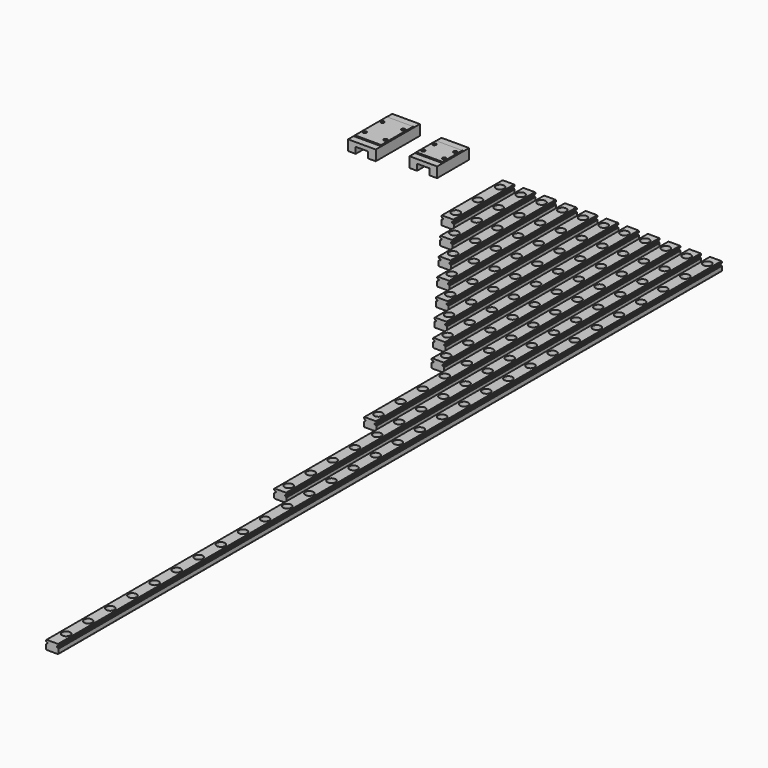
from build123d import *

# Parameters (mm, degrees)
F1_DEPTH           = 55
F2_DEPTH           = 75
F3_DEPTH           = 95
F4_DEPTH           = 115
F5_DEPTH           = 135
F6_DEPTH           = 155
F7_DEPTH           = 175
F8_DEPTH           = 195
F9_DEPTH           = 275
F10_DEPTH          = 375
F11_DEPTH          = 600
F13_D              = 3.5
F13_CBORE_D        = 6
F13_CBORE_DEPTH    = 3.5
F13_2_D            = 3.5
F13_2_CBORE_D      = 6
F13_2_CBORE_DEPTH  = 3.5
F13_3_D            = 3.5
F13_3_CBORE_D      = 6
F13_3_CBORE_DEPTH  = 3.5
F13_4_D            = 3.5
F13_4_CBORE_D      = 6
F13_4_CBORE_DEPTH  = 3.5
F13_5_D            = 3.5
F13_5_CBORE_D      = 6
F13_5_CBORE_DEPTH  = 3.5
F13_6_D            = 3.5
F13_6_CBORE_D      = 6
F13_6_CBORE_DEPTH  = 3.5
F13_7_D            = 3.5
F13_7_CBORE_D      = 6
F13_7_CBORE_DEPTH  = 3.5
F13_8_D            = 3.5
F13_8_CBORE_D      = 6
F13_8_CBORE_DEPTH  = 3.5
F13_9_D            = 3.5
F13_9_CBORE_D      = 6
F13_9_CBORE_DEPTH  = 3.5
F13_10_D           = 3.5
F13_10_CBORE_D     = 6
F13_10_CBORE_DEPTH = 3.5
F14_D              = 3.5
F14_CBORE_D        = 6
F14_CBORE_DEPTH    = 3.5
F16_DEPTH          = 9.45
F18_DEPTH          = 5
F19_DEPTH          = 14.95
F21_DEPTH          = 5
F23_D              = 2.5
F23_DEPTH          = 4.1
F23_TIP            = 0.7510757738
F23_2_D            = 2.5
F23_2_DEPTH        = 4.1
F23_2_TIP          = 0.7510757738
F25_SIZE           = 0.49999


# Not quite as in the source:
# - a fillet or chamfer is up to 0.001 mm smaller than in the source, because OpenCascade refuses the exact size


with BuildPart() as f1:
    # F0 (on Front) → F1 (new body)
    with BuildSketch(Plane.XZ):
        with BuildLine():
            Line((-4.1464466094, -3.25), (4.1464466094, -3.25))
            Line((4.1464466094, -3.25), (4.5, -2.8964466094))
            Line((4.5, -2.8964466094), (4.5, 0.2817541634))
            ThreePointArc((4.5, 0.2817541634), (4.1012202029, 0.4890238013), (3.833484861, 0.85))
            Line((3.833484861, 0.85), (3.3, 0.85))
            Line((3.3, 0.85), (3.3, 1.65))
            Line((3.3, 1.65), (3.833484861, 1.65))
            ThreePointArc((3.833484861, 1.65), (4.1012202029, 2.0109761987), (4.5, 2.2182458366))
            Line((4.5, 2.2182458366), (4.5, 2.8964466094))
            Line((4.5, 2.8964466094), (4.1464466094, 3.25))
            Line((4.1464466094, 3.25), (-4.1464466094, 3.25))
            Line((-4.1464466094, 3.25), (-4.5, 2.8964466094))
            Line((-4.5, 2.8964466094), (-4.5, 2.2182458366))
            ThreePointArc((-4.5, 2.2182458366), (-4.1012202029, 2.0109761987), (-3.833484861, 1.65))
            Line((-3.833484861, 1.65), (-3.3, 1.65))
            Line((-3.3, 1.65), (-3.3, 0.85))
            Line((-3.3, 0.85), (-3.833484861, 0.85))
            ThreePointArc((-3.833484861, 0.85), (-4.1012202029, 0.4890238013), (-4.5, 0.2817541634))
            Line((-4.5, 0.2817541634), (-4.5, -2.8964466094))
            Line((-4.5, -2.8964466094), (-4.1464466094, -3.25))
        make_face()
    extrude(amount=F1_DEPTH)

    # F13 (through all)
    with Locations(Plane.XY.offset(3.25)):
        with Locations((75, -7.5), (135, -47.5), (15, -47.5), (60, -7.5), (90, -27.5), (90, -47.5), (120, -27.5), (30, -7.5), (105, -7.5), (30, -47.5), (0, -47.5), (75, -47.5), (45, -7.5), (90, -7.5), (120, -47.5), (105, -27.5), (15, -7.5), (105, -47.5), (75, -27.5), (135, -27.5), (45, -47.5), (0, -7.5), (60, -47.5), (30, -27.5), (120, -7.5), (45, -27.5), (135, -7.5), (60, -27.5), (0, -27.5), (15, -27.5), (135, -67.5), (30, -67.5), (120, -67.5), (45, -67.5), (15, -67.5), (105, -67.5), (60, -67.5), (75, -67.5), (90, -67.5), (30, -87.5), (45, -87.5), (75, -87.5), (60, -87.5), (105, -87.5), (90, -87.5), (135, -87.5), (120, -87.5), (75, -107.5), (45, -107.5), (60, -107.5), (135, -107.5), (105, -107.5), (120, -107.5), (90, -107.5), (135, -127.5), (105, -127.5), (120, -127.5), (60, -127.5), (75, -127.5), (90, -127.5), (75, -147.5), (90, -147.5), (120, -147.5), (105, -147.5), (135, -147.5), (90, -167.5), (105, -167.5), (135, -167.5), (120, -167.5), (135, -187.5), (105, -187.5), (120, -187.5), (120, -227.5), (135, -267.5), (135, -227.5), (120, -267.5), (120, -207.5), (135, -207.5), (135, -247.5), (120, -247.5), (135, -307.5), (135, -347.5), (135, -367.5), (135, -327.5), (135, -287.5)):
            CounterBoreHole(F13_D / 2, F13_CBORE_D / 2, F13_CBORE_DEPTH)


with BuildPart() as f2:
    # F0 (on Front) → F2 (new body)
    with BuildSketch(Plane.XZ):
        with BuildLine():
            Line((10.5, 0.2817541634), (10.5, -2.8964466094))
            Line((10.5, -2.8964466094), (10.8535533906, -3.25))
            Line((10.8535533906, -3.25), (19.1464466094, -3.25))
            Line((19.1464466094, -3.25), (19.5, -2.8964466094))
            Line((19.5, -2.8964466094), (19.5, 0.2817541634))
            ThreePointArc((19.5, 0.2817541634), (19.1012202029, 0.4890238013), (18.833484861, 0.85))
            Line((18.833484861, 0.85), (18.3, 0.85))
            Line((18.3, 0.85), (18.3, 1.65))
            Line((18.3, 1.65), (18.833484861, 1.65))
            ThreePointArc((18.833484861, 1.65), (19.1012202029, 2.0109761987), (19.5, 2.2182458366))
            Line((19.5, 2.2182458366), (19.5, 2.8964466094))
            Line((19.5, 2.8964466094), (19.1464466094, 3.25))
            Line((19.1464466094, 3.25), (10.8535533906, 3.25))
            Line((10.8535533906, 3.25), (10.5, 2.8964466094))
            Line((10.5, 2.8964466094), (10.5, 2.2182458366))
            ThreePointArc((10.5, 2.2182458366), (10.8987797971, 2.0109761987), (11.166515139, 1.65))
            Line((11.166515139, 1.65), (11.7, 1.65))
            Line((11.7, 1.65), (11.7, 0.85))
            Line((11.7, 0.85), (11.166515139, 0.85))
            ThreePointArc((11.166515139, 0.85), (10.8987797971, 0.4890238013), (10.5, 0.2817541634))
        make_face()
    extrude(amount=F2_DEPTH)

    # F13#2 (through all)
    with Locations(Plane.XY.offset(3.25)):
        with Locations((75, -7.5), (135, -47.5), (15, -47.5), (60, -7.5), (90, -27.5), (90, -47.5), (120, -27.5), (30, -7.5), (105, -7.5), (30, -47.5), (0, -47.5), (75, -47.5), (45, -7.5), (90, -7.5), (120, -47.5), (105, -27.5), (15, -7.5), (105, -47.5), (75, -27.5), (135, -27.5), (45, -47.5), (0, -7.5), (60, -47.5), (30, -27.5), (120, -7.5), (45, -27.5), (135, -7.5), (60, -27.5), (0, -27.5), (15, -27.5), (135, -67.5), (30, -67.5), (120, -67.5), (45, -67.5), (15, -67.5), (105, -67.5), (60, -67.5), (75, -67.5), (90, -67.5), (30, -87.5), (45, -87.5), (75, -87.5), (60, -87.5), (105, -87.5), (90, -87.5), (135, -87.5), (120, -87.5), (75, -107.5), (45, -107.5), (60, -107.5), (135, -107.5), (105, -107.5), (120, -107.5), (90, -107.5), (135, -127.5), (105, -127.5), (120, -127.5), (60, -127.5), (75, -127.5), (90, -127.5), (75, -147.5), (90, -147.5), (120, -147.5), (105, -147.5), (135, -147.5), (90, -167.5), (105, -167.5), (135, -167.5), (120, -167.5), (135, -187.5), (105, -187.5), (120, -187.5), (120, -227.5), (135, -267.5), (135, -227.5), (120, -267.5), (120, -207.5), (135, -207.5), (135, -247.5), (120, -247.5), (135, -307.5), (135, -347.5), (135, -367.5), (135, -327.5), (135, -287.5)):
            CounterBoreHole(F13_2_D / 2, F13_2_CBORE_D / 2, F13_2_CBORE_DEPTH)


with BuildPart() as f3:
    # F0 (on Front) → F3 (new body)
    with BuildSketch(Plane.XZ):
        with BuildLine():
            Line((25.5, 0.2817541634), (25.5, -2.8964466094))
            Line((25.5, -2.8964466094), (25.8535533906, -3.25))
            Line((25.8535533906, -3.25), (34.1464466094, -3.25))
            Line((34.1464466094, -3.25), (34.5, -2.8964466094))
            Line((34.5, -2.8964466094), (34.5, 0.2817541634))
            ThreePointArc((34.5, 0.2817541634), (34.1012202029, 0.4890238013), (33.833484861, 0.85))
            Line((33.833484861, 0.85), (33.3, 0.85))
            Line((33.3, 0.85), (33.3, 1.65))
            Line((33.3, 1.65), (33.833484861, 1.65))
            ThreePointArc((33.833484861, 1.65), (34.1012202029, 2.0109761987), (34.5, 2.2182458366))
            Line((34.5, 2.2182458366), (34.5, 2.8964466094))
            Line((34.5, 2.8964466094), (34.1464466094, 3.25))
            Line((34.1464466094, 3.25), (25.8535533906, 3.25))
            Line((25.8535533906, 3.25), (25.5, 2.8964466094))
            Line((25.5, 2.8964466094), (25.5, 2.2182458366))
            ThreePointArc((25.5, 2.2182458366), (25.8987797971, 2.0109761987), (26.166515139, 1.65))
            Line((26.166515139, 1.65), (26.7, 1.65))
            Line((26.7, 1.65), (26.7, 0.85))
            Line((26.7, 0.85), (26.166515139, 0.85))
            ThreePointArc((26.166515139, 0.85), (25.8987797971, 0.4890238013), (25.5, 0.2817541634))
        make_face()
    extrude(amount=F3_DEPTH)

    # F13#3 (through all)
    with Locations(Plane.XY.offset(3.25)):
        with Locations((75, -7.5), (135, -47.5), (15, -47.5), (60, -7.5), (90, -27.5), (90, -47.5), (120, -27.5), (30, -7.5), (105, -7.5), (30, -47.5), (0, -47.5), (75, -47.5), (45, -7.5), (90, -7.5), (120, -47.5), (105, -27.5), (15, -7.5), (105, -47.5), (75, -27.5), (135, -27.5), (45, -47.5), (0, -7.5), (60, -47.5), (30, -27.5), (120, -7.5), (45, -27.5), (135, -7.5), (60, -27.5), (0, -27.5), (15, -27.5), (135, -67.5), (30, -67.5), (120, -67.5), (45, -67.5), (15, -67.5), (105, -67.5), (60, -67.5), (75, -67.5), (90, -67.5), (30, -87.5), (45, -87.5), (75, -87.5), (60, -87.5), (105, -87.5), (90, -87.5), (135, -87.5), (120, -87.5), (75, -107.5), (45, -107.5), (60, -107.5), (135, -107.5), (105, -107.5), (120, -107.5), (90, -107.5), (135, -127.5), (105, -127.5), (120, -127.5), (60, -127.5), (75, -127.5), (90, -127.5), (75, -147.5), (90, -147.5), (120, -147.5), (105, -147.5), (135, -147.5), (90, -167.5), (105, -167.5), (135, -167.5), (120, -167.5), (135, -187.5), (105, -187.5), (120, -187.5), (120, -227.5), (135, -267.5), (135, -227.5), (120, -267.5), (120, -207.5), (135, -207.5), (135, -247.5), (120, -247.5), (135, -307.5), (135, -347.5), (135, -367.5), (135, -327.5), (135, -287.5)):
            CounterBoreHole(F13_3_D / 2, F13_3_CBORE_D / 2, F13_3_CBORE_DEPTH)


with BuildPart() as f4:
    # F0 (on Front) → F4 (new body)
    with BuildSketch(Plane.XZ):
        with BuildLine():
            Line((40.5, 0.2817541634), (40.5, -2.8964466094))
            Line((40.5, -2.8964466094), (40.8535533906, -3.25))
            Line((40.8535533906, -3.25), (49.1464466094, -3.25))
            Line((49.1464466094, -3.25), (49.5, -2.8964466094))
            Line((49.5, -2.8964466094), (49.5, 0.2817541634))
            ThreePointArc((49.5, 0.2817541634), (49.1012202029, 0.4890238013), (48.833484861, 0.85))
            Line((48.833484861, 0.85), (48.3, 0.85))
            Line((48.3, 0.85), (48.3, 1.65))
            Line((48.3, 1.65), (48.833484861, 1.65))
            ThreePointArc((48.833484861, 1.65), (49.1012202029, 2.0109761987), (49.5, 2.2182458366))
            Line((49.5, 2.2182458366), (49.5, 2.8964466094))
            Line((49.5, 2.8964466094), (49.1464466094, 3.25))
            Line((49.1464466094, 3.25), (40.8535533906, 3.25))
            Line((40.8535533906, 3.25), (40.5, 2.8964466094))
            Line((40.5, 2.8964466094), (40.5, 2.2182458366))
            ThreePointArc((40.5, 2.2182458366), (40.8987797971, 2.0109761987), (41.166515139, 1.65))
            Line((41.166515139, 1.65), (41.7, 1.65))
            Line((41.7, 1.65), (41.7, 0.85))
            Line((41.7, 0.85), (41.166515139, 0.85))
            ThreePointArc((41.166515139, 0.85), (40.8987797971, 0.4890238013), (40.5, 0.2817541634))
        make_face()
    extrude(amount=F4_DEPTH)

    # F13#4 (through all)
    with Locations(Plane.XY.offset(3.25)):
        with Locations((75, -7.5), (135, -47.5), (15, -47.5), (60, -7.5), (90, -27.5), (90, -47.5), (120, -27.5), (30, -7.5), (105, -7.5), (30, -47.5), (0, -47.5), (75, -47.5), (45, -7.5), (90, -7.5), (120, -47.5), (105, -27.5), (15, -7.5), (105, -47.5), (75, -27.5), (135, -27.5), (45, -47.5), (0, -7.5), (60, -47.5), (30, -27.5), (120, -7.5), (45, -27.5), (135, -7.5), (60, -27.5), (0, -27.5), (15, -27.5), (135, -67.5), (30, -67.5), (120, -67.5), (45, -67.5), (15, -67.5), (105, -67.5), (60, -67.5), (75, -67.5), (90, -67.5), (30, -87.5), (45, -87.5), (75, -87.5), (60, -87.5), (105, -87.5), (90, -87.5), (135, -87.5), (120, -87.5), (75, -107.5), (45, -107.5), (60, -107.5), (135, -107.5), (105, -107.5), (120, -107.5), (90, -107.5), (135, -127.5), (105, -127.5), (120, -127.5), (60, -127.5), (75, -127.5), (90, -127.5), (75, -147.5), (90, -147.5), (120, -147.5), (105, -147.5), (135, -147.5), (90, -167.5), (105, -167.5), (135, -167.5), (120, -167.5), (135, -187.5), (105, -187.5), (120, -187.5), (120, -227.5), (135, -267.5), (135, -227.5), (120, -267.5), (120, -207.5), (135, -207.5), (135, -247.5), (120, -247.5), (135, -307.5), (135, -347.5), (135, -367.5), (135, -327.5), (135, -287.5)):
            CounterBoreHole(F13_4_D / 2, F13_4_CBORE_D / 2, F13_4_CBORE_DEPTH)


with BuildPart() as f5:
    # F0 (on Front) → F5 (new body)
    with BuildSketch(Plane.XZ):
        with BuildLine():
            Line((55.5, 0.2817541634), (55.5, -2.8964466094))
            Line((55.5, -2.8964466094), (55.8535533906, -3.25))
            Line((55.8535533906, -3.25), (64.1464466094, -3.25))
            Line((64.1464466094, -3.25), (64.5, -2.8964466094))
            Line((64.5, -2.8964466094), (64.5, 0.2817541634))
            ThreePointArc((64.5, 0.2817541634), (64.1012202029, 0.4890238013), (63.833484861, 0.85))
            Line((63.833484861, 0.85), (63.3, 0.85))
            Line((63.3, 0.85), (63.3, 1.65))
            Line((63.3, 1.65), (63.833484861, 1.65))
            ThreePointArc((63.833484861, 1.65), (64.1012202029, 2.0109761987), (64.5, 2.2182458366))
            Line((64.5, 2.2182458366), (64.5, 2.8964466094))
            Line((64.5, 2.8964466094), (64.1464466094, 3.25))
            Line((64.1464466094, 3.25), (55.8535533906, 3.25))
            Line((55.8535533906, 3.25), (55.5, 2.8964466094))
            Line((55.5, 2.8964466094), (55.5, 2.2182458366))
            ThreePointArc((55.5, 2.2182458366), (55.8987797971, 2.0109761987), (56.166515139, 1.65))
            Line((56.166515139, 1.65), (56.7, 1.65))
            Line((56.7, 1.65), (56.7, 0.85))
            Line((56.7, 0.85), (56.166515139, 0.85))
            ThreePointArc((56.166515139, 0.85), (55.8987797971, 0.4890238013), (55.5, 0.2817541634))
        make_face()
    extrude(amount=F5_DEPTH)

    # F13#5 (through all)
    with Locations(Plane.XY.offset(3.25)):
        with Locations((75, -7.5), (135, -47.5), (15, -47.5), (60, -7.5), (90, -27.5), (90, -47.5), (120, -27.5), (30, -7.5), (105, -7.5), (30, -47.5), (0, -47.5), (75, -47.5), (45, -7.5), (90, -7.5), (120, -47.5), (105, -27.5), (15, -7.5), (105, -47.5), (75, -27.5), (135, -27.5), (45, -47.5), (0, -7.5), (60, -47.5), (30, -27.5), (120, -7.5), (45, -27.5), (135, -7.5), (60, -27.5), (0, -27.5), (15, -27.5), (135, -67.5), (30, -67.5), (120, -67.5), (45, -67.5), (15, -67.5), (105, -67.5), (60, -67.5), (75, -67.5), (90, -67.5), (30, -87.5), (45, -87.5), (75, -87.5), (60, -87.5), (105, -87.5), (90, -87.5), (135, -87.5), (120, -87.5), (75, -107.5), (45, -107.5), (60, -107.5), (135, -107.5), (105, -107.5), (120, -107.5), (90, -107.5), (135, -127.5), (105, -127.5), (120, -127.5), (60, -127.5), (75, -127.5), (90, -127.5), (75, -147.5), (90, -147.5), (120, -147.5), (105, -147.5), (135, -147.5), (90, -167.5), (105, -167.5), (135, -167.5), (120, -167.5), (135, -187.5), (105, -187.5), (120, -187.5), (120, -227.5), (135, -267.5), (135, -227.5), (120, -267.5), (120, -207.5), (135, -207.5), (135, -247.5), (120, -247.5), (135, -307.5), (135, -347.5), (135, -367.5), (135, -327.5), (135, -287.5)):
            CounterBoreHole(F13_5_D / 2, F13_5_CBORE_D / 2, F13_5_CBORE_DEPTH)


with BuildPart() as f6:
    # F0 (on Front) → F6 (new body)
    with BuildSketch(Plane.XZ):
        with BuildLine():
            Line((70.5, 0.2817541634), (70.5, -2.8964466094))
            Line((70.5, -2.8964466094), (70.8535533906, -3.25))
            Line((70.8535533906, -3.25), (79.1464466094, -3.25))
            Line((79.1464466094, -3.25), (79.5, -2.8964466094))
            Line((79.5, -2.8964466094), (79.5, 0.2817541634))
            ThreePointArc((79.5, 0.2817541634), (79.1012202029, 0.4890238013), (78.833484861, 0.85))
            Line((78.833484861, 0.85), (78.3, 0.85))
            Line((78.3, 0.85), (78.3, 1.65))
            Line((78.3, 1.65), (78.833484861, 1.65))
            ThreePointArc((78.833484861, 1.65), (79.1012202029, 2.0109761987), (79.5, 2.2182458366))
            Line((79.5, 2.2182458366), (79.5, 2.8964466094))
            Line((79.5, 2.8964466094), (79.1464466094, 3.25))
            Line((79.1464466094, 3.25), (70.8535533906, 3.25))
            Line((70.8535533906, 3.25), (70.5, 2.8964466094))
            Line((70.5, 2.8964466094), (70.5, 2.2182458366))
            ThreePointArc((70.5, 2.2182458366), (70.8987797971, 2.0109761987), (71.166515139, 1.65))
            Line((71.166515139, 1.65), (71.7, 1.65))
            Line((71.7, 1.65), (71.7, 0.85))
            Line((71.7, 0.85), (71.166515139, 0.85))
            ThreePointArc((71.166515139, 0.85), (70.8987797971, 0.4890238013), (70.5, 0.2817541634))
        make_face()
    extrude(amount=F6_DEPTH)

    # F13#6 (through all)
    with Locations(Plane.XY.offset(3.25)):
        with Locations((75, -7.5), (135, -47.5), (15, -47.5), (60, -7.5), (90, -27.5), (90, -47.5), (120, -27.5), (30, -7.5), (105, -7.5), (30, -47.5), (0, -47.5), (75, -47.5), (45, -7.5), (90, -7.5), (120, -47.5), (105, -27.5), (15, -7.5), (105, -47.5), (75, -27.5), (135, -27.5), (45, -47.5), (0, -7.5), (60, -47.5), (30, -27.5), (120, -7.5), (45, -27.5), (135, -7.5), (60, -27.5), (0, -27.5), (15, -27.5), (135, -67.5), (30, -67.5), (120, -67.5), (45, -67.5), (15, -67.5), (105, -67.5), (60, -67.5), (75, -67.5), (90, -67.5), (30, -87.5), (45, -87.5), (75, -87.5), (60, -87.5), (105, -87.5), (90, -87.5), (135, -87.5), (120, -87.5), (75, -107.5), (45, -107.5), (60, -107.5), (135, -107.5), (105, -107.5), (120, -107.5), (90, -107.5), (135, -127.5), (105, -127.5), (120, -127.5), (60, -127.5), (75, -127.5), (90, -127.5), (75, -147.5), (90, -147.5), (120, -147.5), (105, -147.5), (135, -147.5), (90, -167.5), (105, -167.5), (135, -167.5), (120, -167.5), (135, -187.5), (105, -187.5), (120, -187.5), (120, -227.5), (135, -267.5), (135, -227.5), (120, -267.5), (120, -207.5), (135, -207.5), (135, -247.5), (120, -247.5), (135, -307.5), (135, -347.5), (135, -367.5), (135, -327.5), (135, -287.5)):
            CounterBoreHole(F13_6_D / 2, F13_6_CBORE_D / 2, F13_6_CBORE_DEPTH)


with BuildPart() as f7:
    # F0 (on Front) → F7 (new body)
    with BuildSketch(Plane.XZ):
        with BuildLine():
            Line((85.5, 0.2817541634), (85.5, -2.8964466094))
            Line((85.5, -2.8964466094), (85.8535533906, -3.25))
            Line((85.8535533906, -3.25), (94.1464466094, -3.25))
            Line((94.1464466094, -3.25), (94.5, -2.8964466094))
            Line((94.5, -2.8964466094), (94.5, 0.2817541634))
            ThreePointArc((94.5, 0.2817541634), (94.1012202029, 0.4890238013), (93.833484861, 0.85))
            Line((93.833484861, 0.85), (93.3, 0.85))
            Line((93.3, 0.85), (93.3, 1.65))
            Line((93.3, 1.65), (93.833484861, 1.65))
            ThreePointArc((93.833484861, 1.65), (94.1012202029, 2.0109761987), (94.5, 2.2182458366))
            Line((94.5, 2.2182458366), (94.5, 2.8964466094))
            Line((94.5, 2.8964466094), (94.1464466094, 3.25))
            Line((94.1464466094, 3.25), (85.8535533906, 3.25))
            Line((85.8535533906, 3.25), (85.5, 2.8964466094))
            Line((85.5, 2.8964466094), (85.5, 2.2182458366))
            ThreePointArc((85.5, 2.2182458366), (85.8987797971, 2.0109761987), (86.166515139, 1.65))
            Line((86.166515139, 1.65), (86.7, 1.65))
            Line((86.7, 1.65), (86.7, 0.85))
            Line((86.7, 0.85), (86.166515139, 0.85))
            ThreePointArc((86.166515139, 0.85), (85.8987797971, 0.4890238013), (85.5, 0.2817541634))
        make_face()
    extrude(amount=F7_DEPTH)

    # F13#7 (through all)
    with Locations(Plane.XY.offset(3.25)):
        with Locations((75, -7.5), (135, -47.5), (15, -47.5), (60, -7.5), (90, -27.5), (90, -47.5), (120, -27.5), (30, -7.5), (105, -7.5), (30, -47.5), (0, -47.5), (75, -47.5), (45, -7.5), (90, -7.5), (120, -47.5), (105, -27.5), (15, -7.5), (105, -47.5), (75, -27.5), (135, -27.5), (45, -47.5), (0, -7.5), (60, -47.5), (30, -27.5), (120, -7.5), (45, -27.5), (135, -7.5), (60, -27.5), (0, -27.5), (15, -27.5), (135, -67.5), (30, -67.5), (120, -67.5), (45, -67.5), (15, -67.5), (105, -67.5), (60, -67.5), (75, -67.5), (90, -67.5), (30, -87.5), (45, -87.5), (75, -87.5), (60, -87.5), (105, -87.5), (90, -87.5), (135, -87.5), (120, -87.5), (75, -107.5), (45, -107.5), (60, -107.5), (135, -107.5), (105, -107.5), (120, -107.5), (90, -107.5), (135, -127.5), (105, -127.5), (120, -127.5), (60, -127.5), (75, -127.5), (90, -127.5), (75, -147.5), (90, -147.5), (120, -147.5), (105, -147.5), (135, -147.5), (90, -167.5), (105, -167.5), (135, -167.5), (120, -167.5), (135, -187.5), (105, -187.5), (120, -187.5), (120, -227.5), (135, -267.5), (135, -227.5), (120, -267.5), (120, -207.5), (135, -207.5), (135, -247.5), (120, -247.5), (135, -307.5), (135, -347.5), (135, -367.5), (135, -327.5), (135, -287.5)):
            CounterBoreHole(F13_7_D / 2, F13_7_CBORE_D / 2, F13_7_CBORE_DEPTH)


with BuildPart() as f8:
    # F0 (on Front) → F8 (new body)
    with BuildSketch(Plane.XZ):
        with BuildLine():
            Line((100.5, 0.2817541634), (100.5, -2.8964466094))
            Line((100.5, -2.8964466094), (100.8535533906, -3.25))
            Line((100.8535533906, -3.25), (109.1464466094, -3.25))
            Line((109.1464466094, -3.25), (109.5, -2.8964466094))
            Line((109.5, -2.8964466094), (109.5, 0.2817541634))
            ThreePointArc((109.5, 0.2817541634), (109.1012202029, 0.4890238013), (108.833484861, 0.85))
            Line((108.833484861, 0.85), (108.3, 0.85))
            Line((108.3, 0.85), (108.3, 1.65))
            Line((108.3, 1.65), (108.833484861, 1.65))
            ThreePointArc((108.833484861, 1.65), (109.1012202029, 2.0109761987), (109.5, 2.2182458366))
            Line((109.5, 2.2182458366), (109.5, 2.8964466094))
            Line((109.5, 2.8964466094), (109.1464466094, 3.25))
            Line((109.1464466094, 3.25), (100.8535533906, 3.25))
            Line((100.8535533906, 3.25), (100.5, 2.8964466094))
            Line((100.5, 2.8964466094), (100.5, 2.2182458366))
            ThreePointArc((100.5, 2.2182458366), (100.8987797971, 2.0109761987), (101.166515139, 1.65))
            Line((101.166515139, 1.65), (101.7, 1.65))
            Line((101.7, 1.65), (101.7, 0.85))
            Line((101.7, 0.85), (101.166515139, 0.85))
            ThreePointArc((101.166515139, 0.85), (100.8987797971, 0.4890238013), (100.5, 0.2817541634))
        make_face()
    extrude(amount=F8_DEPTH)

    # F13#8 (through all)
    with Locations(Plane.XY.offset(3.25)):
        with Locations((75, -7.5), (135, -47.5), (15, -47.5), (60, -7.5), (90, -27.5), (90, -47.5), (120, -27.5), (30, -7.5), (105, -7.5), (30, -47.5), (0, -47.5), (75, -47.5), (45, -7.5), (90, -7.5), (120, -47.5), (105, -27.5), (15, -7.5), (105, -47.5), (75, -27.5), (135, -27.5), (45, -47.5), (0, -7.5), (60, -47.5), (30, -27.5), (120, -7.5), (45, -27.5), (135, -7.5), (60, -27.5), (0, -27.5), (15, -27.5), (135, -67.5), (30, -67.5), (120, -67.5), (45, -67.5), (15, -67.5), (105, -67.5), (60, -67.5), (75, -67.5), (90, -67.5), (30, -87.5), (45, -87.5), (75, -87.5), (60, -87.5), (105, -87.5), (90, -87.5), (135, -87.5), (120, -87.5), (75, -107.5), (45, -107.5), (60, -107.5), (135, -107.5), (105, -107.5), (120, -107.5), (90, -107.5), (135, -127.5), (105, -127.5), (120, -127.5), (60, -127.5), (75, -127.5), (90, -127.5), (75, -147.5), (90, -147.5), (120, -147.5), (105, -147.5), (135, -147.5), (90, -167.5), (105, -167.5), (135, -167.5), (120, -167.5), (135, -187.5), (105, -187.5), (120, -187.5), (120, -227.5), (135, -267.5), (135, -227.5), (120, -267.5), (120, -207.5), (135, -207.5), (135, -247.5), (120, -247.5), (135, -307.5), (135, -347.5), (135, -367.5), (135, -327.5), (135, -287.5)):
            CounterBoreHole(F13_8_D / 2, F13_8_CBORE_D / 2, F13_8_CBORE_DEPTH)


with BuildPart() as f9:
    # F0 (on Front) → F9 (new body)
    with BuildSketch(Plane.XZ):
        with BuildLine():
            Line((115.5, 0.2817541634), (115.5, -2.8964466094))
            Line((115.5, -2.8964466094), (115.8535533906, -3.25))
            Line((115.8535533906, -3.25), (124.1464466094, -3.25))
            Line((124.1464466094, -3.25), (124.5, -2.8964466094))
            Line((124.5, -2.8964466094), (124.5, 0.2817541634))
            ThreePointArc((124.5, 0.2817541634), (124.1012202029, 0.4890238013), (123.833484861, 0.85))
            Line((123.833484861, 0.85), (123.3, 0.85))
            Line((123.3, 0.85), (123.3, 1.65))
            Line((123.3, 1.65), (123.833484861, 1.65))
            ThreePointArc((123.833484861, 1.65), (124.1012202029, 2.0109761987), (124.5, 2.2182458366))
            Line((124.5, 2.2182458366), (124.5, 2.8964466094))
            Line((124.5, 2.8964466094), (124.1464466094, 3.25))
            Line((124.1464466094, 3.25), (115.8535533906, 3.25))
            Line((115.8535533906, 3.25), (115.5, 2.8964466094))
            Line((115.5, 2.8964466094), (115.5, 2.2182458366))
            ThreePointArc((115.5, 2.2182458366), (115.8987797971, 2.0109761987), (116.166515139, 1.65))
            Line((116.166515139, 1.65), (116.7, 1.65))
            Line((116.7, 1.65), (116.7, 0.85))
            Line((116.7, 0.85), (116.166515139, 0.85))
            ThreePointArc((116.166515139, 0.85), (115.8987797971, 0.4890238013), (115.5, 0.2817541634))
        make_face()
    extrude(amount=F9_DEPTH)

    # F13#9 (through all)
    with Locations(Plane.XY.offset(3.25)):
        with Locations((75, -7.5), (135, -47.5), (15, -47.5), (60, -7.5), (90, -27.5), (90, -47.5), (120, -27.5), (30, -7.5), (105, -7.5), (30, -47.5), (0, -47.5), (75, -47.5), (45, -7.5), (90, -7.5), (120, -47.5), (105, -27.5), (15, -7.5), (105, -47.5), (75, -27.5), (135, -27.5), (45, -47.5), (0, -7.5), (60, -47.5), (30, -27.5), (120, -7.5), (45, -27.5), (135, -7.5), (60, -27.5), (0, -27.5), (15, -27.5), (135, -67.5), (30, -67.5), (120, -67.5), (45, -67.5), (15, -67.5), (105, -67.5), (60, -67.5), (75, -67.5), (90, -67.5), (30, -87.5), (45, -87.5), (75, -87.5), (60, -87.5), (105, -87.5), (90, -87.5), (135, -87.5), (120, -87.5), (75, -107.5), (45, -107.5), (60, -107.5), (135, -107.5), (105, -107.5), (120, -107.5), (90, -107.5), (135, -127.5), (105, -127.5), (120, -127.5), (60, -127.5), (75, -127.5), (90, -127.5), (75, -147.5), (90, -147.5), (120, -147.5), (105, -147.5), (135, -147.5), (90, -167.5), (105, -167.5), (135, -167.5), (120, -167.5), (135, -187.5), (105, -187.5), (120, -187.5), (120, -227.5), (135, -267.5), (135, -227.5), (120, -267.5), (120, -207.5), (135, -207.5), (135, -247.5), (120, -247.5), (135, -307.5), (135, -347.5), (135, -367.5), (135, -327.5), (135, -287.5)):
            CounterBoreHole(F13_9_D / 2, F13_9_CBORE_D / 2, F13_9_CBORE_DEPTH)


with BuildPart() as f10:
    # F0 (on Front) → F10 (new body)
    with BuildSketch(Plane.XZ):
        with BuildLine():
            Line((130.5, 0.2817541634), (130.5, -2.8964466094))
            Line((130.5, -2.8964466094), (130.8535533906, -3.25))
            Line((130.8535533906, -3.25), (139.1464466094, -3.25))
            Line((139.1464466094, -3.25), (139.5, -2.8964466094))
            Line((139.5, -2.8964466094), (139.5, 0.2817541634))
            ThreePointArc((139.5, 0.2817541634), (139.1012202029, 0.4890238013), (138.833484861, 0.85))
            Line((138.833484861, 0.85), (138.3, 0.85))
            Line((138.3, 0.85), (138.3, 1.65))
            Line((138.3, 1.65), (138.833484861, 1.65))
            ThreePointArc((138.833484861, 1.65), (139.1012202029, 2.0109761987), (139.5, 2.2182458366))
            Line((139.5, 2.2182458366), (139.5, 2.8964466094))
            Line((139.5, 2.8964466094), (139.1464466094, 3.25))
            Line((139.1464466094, 3.25), (130.8535533906, 3.25))
            Line((130.8535533906, 3.25), (130.5, 2.8964466094))
            Line((130.5, 2.8964466094), (130.5, 2.2182458366))
            ThreePointArc((130.5, 2.2182458366), (130.8987797971, 2.0109761987), (131.166515139, 1.65))
            Line((131.166515139, 1.65), (131.7, 1.65))
            Line((131.7, 1.65), (131.7, 0.85))
            Line((131.7, 0.85), (131.166515139, 0.85))
            ThreePointArc((131.166515139, 0.85), (130.8987797971, 0.4890238013), (130.5, 0.2817541634))
        make_face()
    extrude(amount=F10_DEPTH)

    # F13#10 (through all)
    with Locations(Plane.XY.offset(3.25)):
        with Locations((75, -7.5), (135, -47.5), (15, -47.5), (60, -7.5), (90, -27.5), (90, -47.5), (120, -27.5), (30, -7.5), (105, -7.5), (30, -47.5), (0, -47.5), (75, -47.5), (45, -7.5), (90, -7.5), (120, -47.5), (105, -27.5), (15, -7.5), (105, -47.5), (75, -27.5), (135, -27.5), (45, -47.5), (0, -7.5), (60, -47.5), (30, -27.5), (120, -7.5), (45, -27.5), (135, -7.5), (60, -27.5), (0, -27.5), (15, -27.5), (135, -67.5), (30, -67.5), (120, -67.5), (45, -67.5), (15, -67.5), (105, -67.5), (60, -67.5), (75, -67.5), (90, -67.5), (30, -87.5), (45, -87.5), (75, -87.5), (60, -87.5), (105, -87.5), (90, -87.5), (135, -87.5), (120, -87.5), (75, -107.5), (45, -107.5), (60, -107.5), (135, -107.5), (105, -107.5), (120, -107.5), (90, -107.5), (135, -127.5), (105, -127.5), (120, -127.5), (60, -127.5), (75, -127.5), (90, -127.5), (75, -147.5), (90, -147.5), (120, -147.5), (105, -147.5), (135, -147.5), (90, -167.5), (105, -167.5), (135, -167.5), (120, -167.5), (135, -187.5), (105, -187.5), (120, -187.5), (120, -227.5), (135, -267.5), (135, -227.5), (120, -267.5), (120, -207.5), (135, -207.5), (135, -247.5), (120, -247.5), (135, -307.5), (135, -347.5), (135, -367.5), (135, -327.5), (135, -287.5)):
            CounterBoreHole(F13_10_D / 2, F13_10_CBORE_D / 2, F13_10_CBORE_DEPTH)


with BuildPart() as f11:
    # F0 (on Front) → F11 (new body)
    with BuildSketch(Plane.XZ):
        with BuildLine():
            Line((145.5, 0.2817541634), (145.5, -2.8964466094))
            Line((145.5, -2.8964466094), (145.8535533906, -3.25))
            Line((145.8535533906, -3.25), (154.1464466094, -3.25))
            Line((154.1464466094, -3.25), (154.5, -2.8964466094))
            Line((154.5, -2.8964466094), (154.5, 0.2817541634))
            ThreePointArc((154.5, 0.2817541634), (154.1012202029, 0.4890238013), (153.833484861, 0.85))
            Line((153.833484861, 0.85), (153.3, 0.85))
            Line((153.3, 0.85), (153.3, 1.65))
            Line((153.3, 1.65), (153.833484861, 1.65))
            ThreePointArc((153.833484861, 1.65), (154.1012202029, 2.0109761987), (154.5, 2.2182458366))
            Line((154.5, 2.2182458366), (154.5, 2.8964466094))
            Line((154.5, 2.8964466094), (154.1464466094, 3.25))
            Line((154.1464466094, 3.25), (145.8535533906, 3.25))
            Line((145.8535533906, 3.25), (145.5, 2.8964466094))
            Line((145.5, 2.8964466094), (145.5, 2.2182458366))
            ThreePointArc((145.5, 2.2182458366), (145.8987797971, 2.0109761987), (146.166515139, 1.65))
            Line((146.166515139, 1.65), (146.7, 1.65))
            Line((146.7, 1.65), (146.7, 0.85))
            Line((146.7, 0.85), (146.166515139, 0.85))
            ThreePointArc((146.166515139, 0.85), (145.8987797971, 0.4890238013), (145.5, 0.2817541634))
        make_face()
    extrude(amount=F11_DEPTH)

    # F14 (through all)
    with Locations(Plane.XY.offset(3.25)):
        with Locations((150, -7.5), (150, -487.5), (150, -247.5), (150, -327.5), (150, -667.5), (150, -647.5), (150, -727.5), (150, -567.5), (150, -747.5), (150, -87.5), (150, -167.5), (150, -407.5), (150, -107.5), (150, -27.5), (150, -427.5), (150, -347.5), (150, -267.5), (150, -187.5), (150, -587.5), (150, -507.5), (150, -127.5), (150, -47.5), (150, -447.5), (150, -367.5), (150, -287.5), (150, -207.5), (150, -607.5), (150, -527.5), (150, -767.5), (150, -687.5), (150, -307.5), (150, -227.5), (150, -147.5), (150, -67.5), (150, -627.5), (150, -547.5), (150, -467.5), (150, -387.5), (150, -787.5), (150, -707.5), (150, -847.5), (150, -867.5), (150, -967.5), (150, -887.5), (150, -827.5), (150, -987.5), (150, -907.5), (150, -927.5), (150, -947.5), (150, -807.5)):
            CounterBoreHole(F14_D / 2, F14_CBORE_D / 2, F14_CBORE_DEPTH)


with BuildPart() as f16:
    # F15 (on Front) → F16 (new body)
    with BuildSketch(Plane.XZ):
        with BuildLine():
            Line((-40, 6.25), (-60, 6.25))
            Line((-60, 6.25), (-60, -1.25))
            Line((-60, -1.25), (-54.5, -1.25))
            Line((-54.5, -1.25), (-54.5, 0.25))
            ThreePointArc((-54.5, 0.25), (-55.5, 1.25), (-54.5, 2.25))
            Line((-54.5, 2.25), (-54.5, 3.25))
            Line((-54.5, 3.25), (-50, 3.25))
            Line((-50, 3.25), (-45.5, 3.25))
            Line((-45.5, 3.25), (-45.5, 2.25))
            ThreePointArc((-45.5, 2.25), (-44.5, 1.25), (-45.5, 0.25))
            Line((-45.5, 0.25), (-45.5, -1.25))
            Line((-45.5, -1.25), (-40, -1.25))
            Line((-40, -1.25), (-40, 6.25))
        make_face()
        Polygon((-40, 6.75), (-50, 6.75), (-60, 6.75), (-60, 6.25), (-40, 6.25), align=None)
    extrude(amount=F16_DEPTH)

    # F17 (on face) → F18 (join)
    with BuildSketch(Plane.XZ.offset(9.45)):
        with BuildLine():
            ThreePointArc((-54.5, 2.25), (-55.5, 1.25), (-54.5, 0.25))
            Line((-54.5, 0.25), (-54.5, 2.25))
        make_face()
        with BuildLine():
            Line((-54.5, -1.25), (-54.5, 0.25))
            ThreePointArc((-54.5, 0.25), (-55.5, 1.25), (-54.5, 2.25))
            Line((-54.5, 2.25), (-54.5, 3.25))
            Line((-54.5, 3.25), (-45.5, 3.25))
            Line((-45.5, 3.25), (-45.5, 2.25))
            ThreePointArc((-45.5, 2.25), (-44.5, 1.25), (-45.5, 0.25))
            Line((-45.5, 0.25), (-45.5, -1.25))
            Line((-45.5, -1.25), (-40, -1.25))
            Line((-40, -1.25), (-40, 6.25))
            Line((-40, 6.25), (-60, 6.25))
            Line((-60, 6.25), (-60, -1.25))
            Line((-60, -1.25), (-54.5, -1.25))
        make_face()
        with BuildLine():
            ThreePointArc((-45.5, 0.25), (-44.5, 1.25), (-45.5, 2.25))
            Line((-45.5, 2.25), (-45.5, 0.25))
        make_face()
    extrude(amount=F18_DEPTH)

    # F23
    with Locations(Plane.XY.offset(6.75)):
        with Locations((-57.5, -5), (-42.5, -5), (-82.5, -8), (-97.5, -8)):
            Hole(F23_D / 2, depth=F23_DEPTH)
            with Locations((0, 0, -(F23_DEPTH + F23_TIP / 2))):  # 118° drill point
                Cone(0, F23_D / 2, F23_TIP, mode=Mode.SUBTRACT)



with BuildPart() as f19:
    # F15 (on Front) → F19 (new body)
    with BuildSketch(Plane.XZ):
        with BuildLine():
            Line((-80, 6.25), (-100, 6.25))
            Line((-100, 6.25), (-100, -1.25))
            Line((-100, -1.25), (-94.5, -1.25))
            Line((-94.5, -1.25), (-94.5, 0.25))
            ThreePointArc((-94.5, 0.25), (-95.5, 1.25), (-94.5, 2.25))
            Line((-94.5, 2.25), (-94.5, 3.25))
            Line((-94.5, 3.25), (-90, 3.25))
            Line((-90, 3.25), (-85.5, 3.25))
            Line((-85.5, 3.25), (-85.5, 2.25))
            ThreePointArc((-85.5, 2.25), (-84.5, 1.25), (-85.5, 0.25))
            Line((-85.5, 0.25), (-85.5, -1.25))
            Line((-85.5, -1.25), (-80, -1.25))
            Line((-80, -1.25), (-80, 6.25))
        make_face()
        Polygon((-90, 6.75), (-100, 6.75), (-100, 6.25), (-80, 6.25), (-80, 6.75), align=None)
    extrude(amount=F19_DEPTH)

    # F20 (on face) → F21 (join)
    with BuildSketch(Plane.XZ.offset(14.95)):
        with BuildLine():
            Line((-94.5, -1.25), (-94.5, 0.25))
            ThreePointArc((-94.5, 0.25), (-95.5, 1.25), (-94.5, 2.25))
            Line((-94.5, 2.25), (-94.5, 3.25))
            Line((-94.5, 3.25), (-85.5, 3.25))
            Line((-85.5, 3.25), (-85.5, 2.25))
            ThreePointArc((-85.5, 2.25), (-84.5, 1.25), (-85.5, 0.25))
            Line((-85.5, 0.25), (-85.5, -1.25))
            Line((-85.5, -1.25), (-80, -1.25))
            Line((-80, -1.25), (-80, 6.25))
            Line((-80, 6.25), (-100, 6.25))
            Line((-100, 6.25), (-100, -1.25))
            Line((-100, -1.25), (-94.5, -1.25))
        make_face()
        with BuildLine():
            ThreePointArc((-94.5, 2.25), (-95.5, 1.25), (-94.5, 0.25))
            Line((-94.5, 0.25), (-94.5, 2.25))
        make_face()
        with BuildLine():
            ThreePointArc((-85.5, 0.25), (-84.5, 1.25), (-85.5, 2.25))
            Line((-85.5, 2.25), (-85.5, 0.25))
        make_face()
    extrude(amount=F21_DEPTH)

    # F23#2
    with Locations(Plane.XY.offset(6.75)):
        with Locations((-57.5, -5), (-42.5, -5), (-82.5, -8), (-97.5, -8)):
            Hole(F23_2_D / 2, depth=F23_2_DEPTH)
            with Locations((0, 0, -(F23_2_DEPTH + F23_2_TIP / 2))):  # 118° drill point
                Cone(0, F23_2_D / 2, F23_2_TIP, mode=Mode.SUBTRACT)


with BuildPart() as f16_1:
    add(f16.part)

    add(f19.part)  # F24 merges F19
    # F24: F19, F16 across face
    add(f19.part.mirror(Plane.XZ))
    add(f16.part.mirror(Plane.XZ))

    # F25 (size 0.5 in the source; OpenCascade refuses exactly that, so slightly less here)
    f25_edges = [f16_1.edges().sort_by_distance(p)[0] for p in [
        (-50, -9.45, 6.75),
        (-50, 9.45, 6.75),
        (-40, 0, 6.75),
        (-60, 0, 6.75),
        (-80, 0, 6.75),
        (-90, -14.95, 6.75),
        (-90, 14.95, 6.75),
        (-100, 0, 6.75),
    ]]
    chamfer(f25_edges, length=F25_SIZE)


solid = Compound([f1.part, f2.part, f3.part, f4.part, f5.part, f6.part, f7.part, f8.part, f9.part, f10.part, f11.part, f16_1.part])
